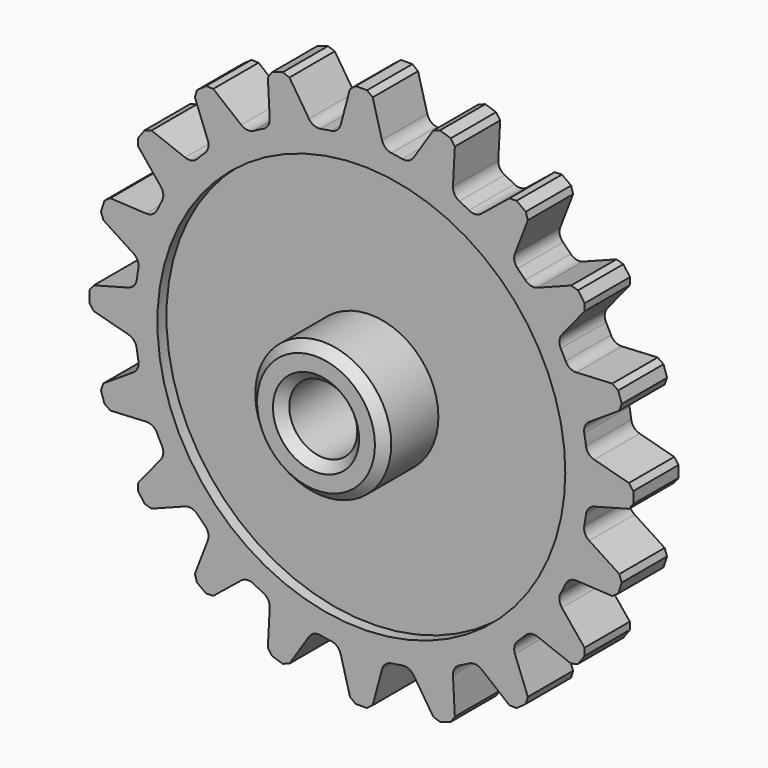
from build123d import *

# Parameters (mm, degrees)
F0_R            = 100
F1_DEPTH        = 25
F3_DEPTH        = 25
F3_COPIES_COUNT = 20
F4_SIZE         = 2
F5_R            = 5
F6_R            = 90
F7_DEPTH        = 5
F8_R            = 30
F9_DEPTH        = 30
F10_R           = 15
F11_DEPTH       = 50.001
F12_SIZE        = 4


# Not quite as in the source:
# - a pattern or mirror of a feature is missing from the dataset's text; its kind, count and spacing are read off the source's solid


with BuildPart() as f1:
    # F0 (on Front) → F1 (new body)
    with BuildSketch(Plane.XZ):
        Circle(F0_R)
    extrude(amount=F1_DEPTH)

    # F2 (on face) → F3 (join)
    with BuildSketch(Plane.XZ.offset(25)):
        with BuildLine():
            Line((9.9931095726, 99.4994359837), (4.5, 120))
            Line((4.5, 120), (-4.5, 120))
            Line((-4.5, 120), (-9.9931095726, 99.4994359837))
            ThreePointArc((-9.9931095726, 99.4994359837), (0, 100), (9.9931095726, 99.4994359837))
        make_face()
    f3 = extrude(amount=-F3_DEPTH)

    # F3_copies: F3 ×20 about axis
    f3_copies_axis = Axis((0, 0, 0), (0, 1, 0))
    for i in range(1, F3_COPIES_COUNT):
        add(f3.rotate(f3_copies_axis, i * 360 / F3_COPIES_COUNT))

    # F4
    f4_edges = [f1.edges().sort_by_distance(p)[0] for p in [
        (4.5, -12.5, 120),
        (-4.5, -12.5, 120),
        (-32.802285, -12.5, 115.517358),
        (-66.893654, -12.5, 99.727073),
        (-74.174807, -12.5, 94.437006),
        (-94.437006, -12.5, 74.174807),
        (-99.727073, -12.5, 66.893654),
        (-112.736205, -12.5, 41.361794),
        (-115.517358, -12.5, 32.802285),
        (-120, -12.5, 4.5),
        (-120, -12.5, -4.5),
        (-115.517358, -12.5, -32.802285),
        (-112.736205, -12.5, -41.361794),
        (-99.727073, -12.5, -66.893654),
        (-94.437006, -12.5, -74.174807),
        (-74.174807, -12.5, -94.437006),
        (-66.893654, -12.5, -99.727073),
        (-41.361794, -12.5, -112.736205),
        (-32.802285, -12.5, -115.517358),
        (-4.5, -12.5, -120),
        (4.5, -12.5, -120),
        (32.802285, -12.5, -115.517358),
        (41.361794, -12.5, -112.736205),
        (66.893654, -12.5, -99.727073),
        (74.174807, -12.5, -94.437006),
        (94.437006, -12.5, -74.174807),
        (99.727073, -12.5, -66.893654),
        (112.736205, -12.5, -41.361794),
        (115.517358, -12.5, -32.802285),
        (120, -12.5, -4.5),
        (120, -12.5, 4.5),
        (115.517358, -12.5, 32.802285),
        (112.736205, -12.5, 41.361794),
        (99.727073, -12.5, 66.893654),
        (94.437006, -12.5, 74.174807),
        (74.174807, -12.5, 94.437006),
        (66.893654, -12.5, 99.727073),
        (41.361794, -12.5, 112.736205),
        (32.802285, -12.5, 115.517358),
        (-41.361794, -12.5, 112.736205),
    ]]
    chamfer(f4_edges, length=F4_SIZE)

    # F5
    f5_edges = [f1.edges().sort_by_distance(p)[0] for p in [
        (-9.99311, -12.5, 99.499436),
        (9.99311, -12.5, 99.499436),
        (21.243005, -12.5, 97.717628),
        (-21.243005, -12.5, 97.717628),
        (40.251029, -12.5, 91.541546),
        (50.399706, -12.5, 86.370537),
        (-40.251029, -12.5, 91.541546),
        (-50.399706, -12.5, 86.370537),
        (66.568897, -12.5, 74.622932),
        (74.622932, -12.5, 66.568897),
        (-66.568897, -12.5, 74.622932),
        (-74.622932, -12.5, 66.568897),
        (86.370537, -12.5, 50.399706),
        (91.541546, -12.5, 40.251029),
        (-86.370537, -12.5, 50.399706),
        (-91.541546, -12.5, 40.251029),
        (97.717628, -12.5, 21.243005),
        (99.499436, -12.5, 9.99311),
        (-97.717628, -12.5, 21.243005),
        (-99.499436, -12.5, 9.99311),
        (99.499436, -12.5, -9.99311),
        (97.717628, -12.5, -21.243005),
        (-99.499436, -12.5, -9.99311),
        (-97.717628, -12.5, -21.243005),
        (91.541546, -12.5, -40.251029),
        (86.370537, -12.5, -50.399706),
        (-91.541546, -12.5, -40.251029),
        (-86.370537, -12.5, -50.399706),
        (74.622932, -12.5, -66.568897),
        (66.568897, -12.5, -74.622932),
        (-74.622932, -12.5, -66.568897),
        (-66.568897, -12.5, -74.622932),
        (50.399706, -12.5, -86.370537),
        (40.251029, -12.5, -91.541546),
        (-50.399706, -12.5, -86.370537),
        (-40.251029, -12.5, -91.541546),
        (21.243005, -12.5, -97.717628),
        (9.99311, -12.5, -99.499436),
        (-21.243005, -12.5, -97.717628),
        (-9.99311, -12.5, -99.499436),
    ]]
    fillet(f5_edges, radius=F5_R)

    # F6 (on face) → F7 (cut)
    with BuildSketch(Plane.XZ.offset(25)):
        Circle(F6_R)
    extrude(amount=-F7_DEPTH, mode=Mode.SUBTRACT)

    # F8 (on face) → F9 (join)
    with BuildSketch(Plane.XZ.offset(20)):
        Circle(F8_R)
    extrude(amount=F9_DEPTH)

    # F10 (on face) → F11 (cut, through all)
    with BuildSketch(Plane.XZ.offset(50)):
        Circle(F10_R)
    extrude(amount=-F11_DEPTH, mode=Mode.SUBTRACT)

    # F12
    f12_edges = [f1.edges().sort_by_distance(p)[0] for p in [
        (-30, -50, 0),
        (-15, -50, 0),
    ]]
    chamfer(f12_edges, length=F12_SIZE)


solid = f1.part
